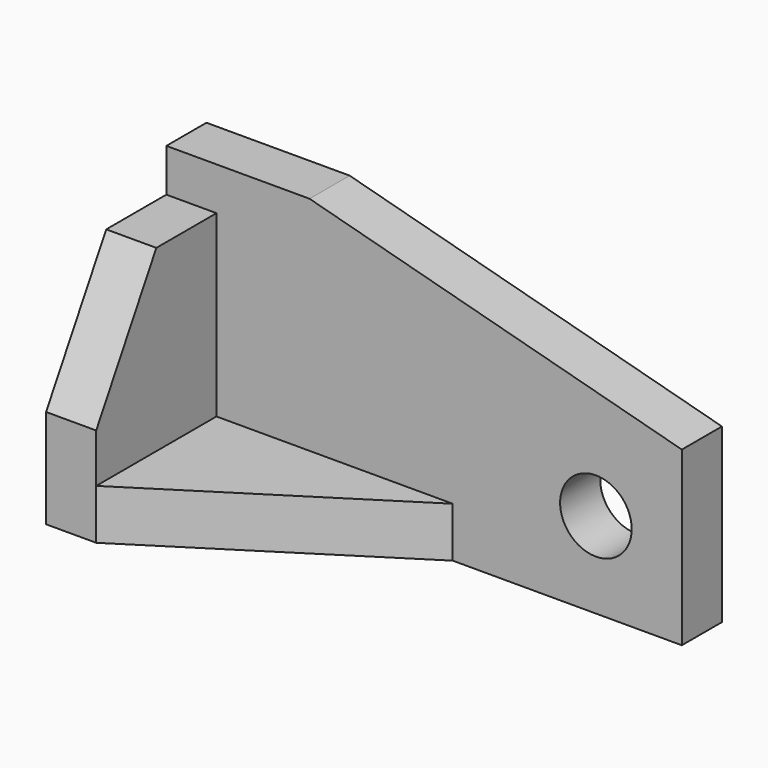
from build123d import *

# Parameters (mm, degrees)
F1_DEPTH = 11.1125
F2_DEPTH = 60.325
F0_W     = 11.1125
F0_H     = 33.3375
F3_DEPTH = 50.8
F6_DEPTH = 11.1125
F7_DEPTH = 11.1125
F4_R     = 7.9375
F8_DEPTH = 11.1125


# Not quite as in the source:
# - a length typed as a fraction of an inch, garbled in the dataset ("3 / 203.2 mm" for 3/8 in), is restored


with BuildPart() as f1:
    # F0 (on Top) → F1 (new body)
    with BuildSketch(Plane.XY):
        Polygon((-46.0375, 11.1125), (-46.0375, -22.225), (6.35, 11.1125), (-25.4, 11.1125), align=None)
    extrude(amount=F1_DEPTH)

    # F0 (on Top) → F2 (join)
    with BuildSketch(Plane.XY):
        Polygon((-57.15, 11.1125), (-46.0375, 11.1125), (-25.4, 11.1125), (-25.4, 22.225), (-57.15, 22.225), align=None)
        Polygon((-25.4, 11.1125), (6.35, 11.1125), (57.15, 11.1125), (57.15, 22.225), (-25.4, 22.225), align=None)
    extrude(amount=F2_DEPTH)

    # F0 (on Top) → F3 (join)
    with BuildSketch(Plane.XY):
        with Locations((-51.59375, -5.55625)):
            Rectangle(F0_W, F0_H)
    extrude(amount=F3_DEPTH)

    # F5 (on face) → F6 (cut)
    with BuildSketch(Plane.YZ.offset(-46.0375)):
        Polygon((-22.225, 50.8), (-22.225, 21.9288781013), (-5.55625, 50.8), align=None)
    extrude(amount=-F6_DEPTH, mode=Mode.SUBTRACT)

    # F4 (on face) → F7 (cut)
    with BuildSketch(Plane.XZ.offset(-11.1125)):
        Polygon((57.15, 60.325), (-25.4, 60.325), (57.15, 38.2057941648), align=None)
    extrude(amount=-F7_DEPTH, mode=Mode.SUBTRACT)

    # F4 (on face) → F8 (cut)
    with BuildSketch(Plane.XZ.offset(-11.1125)):
        with Locations((38.1, 19.05)):
            Circle(F4_R)
    extrude(amount=-F8_DEPTH, mode=Mode.SUBTRACT)


solid = f1.part
